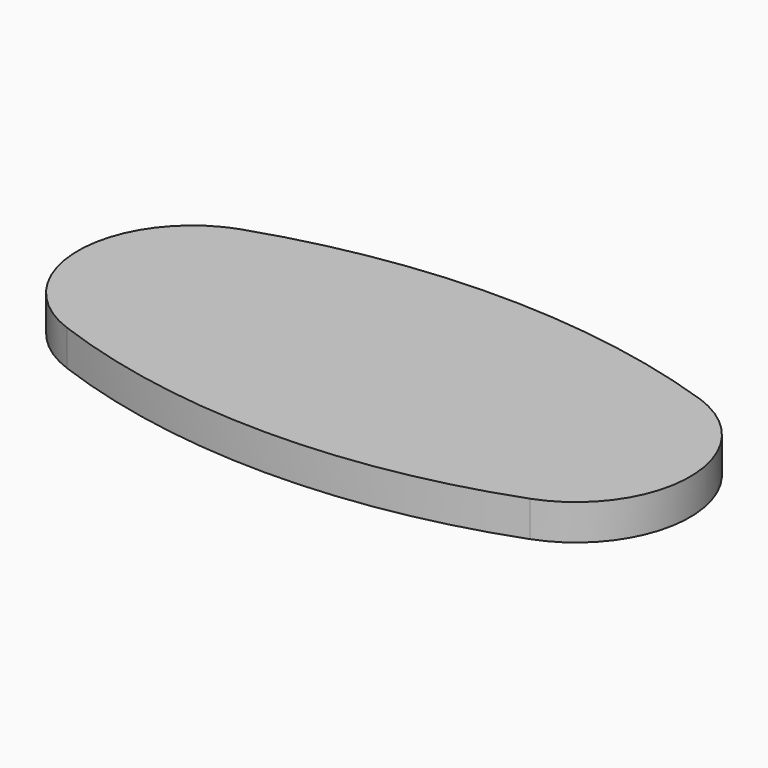
from build123d import *

# Parameters (mm, degrees)
F1_DEPTH = 6.35
F2_R     = 20.32


with BuildPart() as f1:
    # F0 (on Top) → F1 (new body)
    with BuildSketch(Plane.XY):
        with BuildLine():
            ThreePointArc((-76.504804194, 0), (-0.6095990539, -27.2374155304), (75.2856060863, 0))
            ThreePointArc((75.2856060863, 0), (-0.6095990539, 25.123818391), (-76.504804194, 0))
        make_face()
    extrude(amount=F1_DEPTH)

    # F2
    f2_edges = [f1.edges().sort_by_distance(p)[0] for p in [
        (75.285606, 0, 3.175),
        (-76.504804, 0, 3.175),
    ]]
    fillet(f2_edges, radius=F2_R)


solid = f1.part
